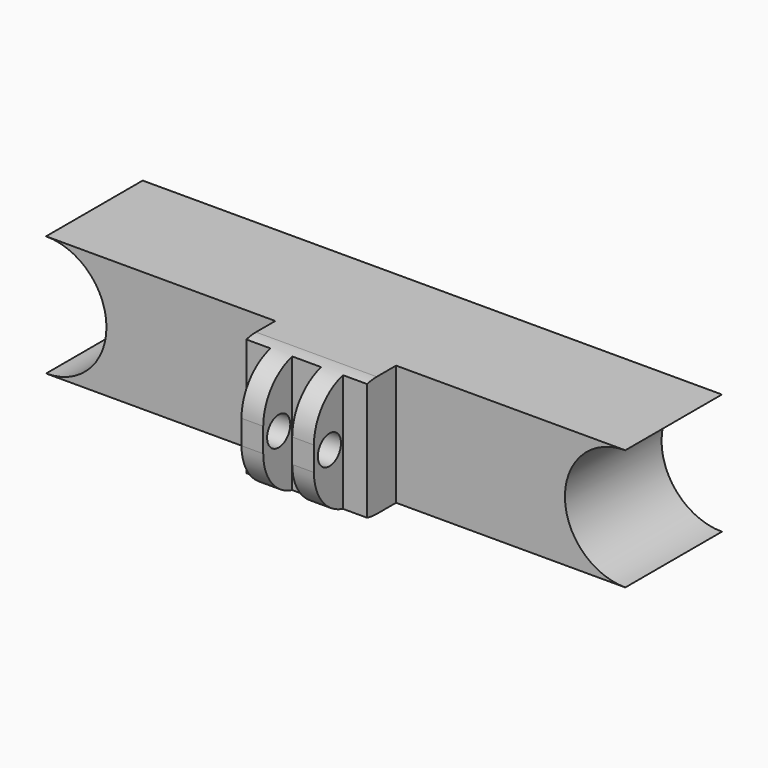
from build123d import *

# Parameters (mm, degrees)
F1_DEPTH  = 25
F2_W      = 50
F2_H      = 50
F3_DEPTH  = 30
F6_W      = 6
F6_H      = 15
F5_W      = 6
F5_H      = 15
F4_W      = 10
F4_H      = 15
F7_DEPTH  = 50.001
F8_F1_R   = 20
F8_F2_R   = 20
F9_R      = 6
F10_DEPTH = 134.901


with BuildPart() as f1:
    # F0 (on Front) → F1 (new body, symmetric)
    with BuildSketch(Plane.XZ):
        with BuildLine():
            Line((-119.9, -25), (119.9, -25))
            ThreePointArc((119.9, -25), (94.9, 0), (119.9, 25))
            Line((119.9, 25), (-119.9, 25))
            ThreePointArc((-119.9, 25), (-94.9, 0), (-119.9, -25))
        make_face()
    extrude(amount=F1_DEPTH, both=True)

    # F2 (on face) → F3 (join)
    with BuildSketch(Plane.XZ.offset(25)):
        Rectangle(F2_W, F2_H)
    extrude(amount=F3_DEPTH)

    # F6 (on face) + F5 (on face) + F4 (on face) → F7 (cut, through all)
    with BuildSketch(Plane(origin=(0, 0, -25), x_dir=(1, 0, 0), z_dir=(0, 0, -1))):
        with Locations((-3, 47.5)):
            Rectangle(F6_W, F6_H)
    with BuildSketch(Plane(origin=(0, 0, -25), x_dir=(1, 0, 0), z_dir=(0, 0, -1))):
        with Locations((3, 47.5)):
            Rectangle(F5_W, F5_H)
    with BuildSketch(Plane(origin=(0, 0, -25), x_dir=(1, 0, 0), z_dir=(0, 0, -1))):
        with Locations((20, 47.5)):
            Rectangle(F4_W, F4_H)
        with Locations((-20, 47.5)):
            Rectangle(F4_W, F4_H)
    extrude(amount=-F7_DEPTH, mode=Mode.SUBTRACT)

    # F8: fillet of radius 20 on 4 edges, made by hand

    # F8_f1
    f8_f1_edges = [f1.edges().sort_by_distance(p)[0] for p in [
        (10.5, -55, 25),
    ]]
    fillet(f8_f1_edges, radius=F8_F1_R)

    # F8_f2
    f8_f2_edges = [f1.edges().sort_by_distance(p)[0] for p in [
        (10.5, -55, -25),
    ]]
    fillet(f8_f2_edges, radius=F8_F2_R)

    # F9 (on face) → F10 (cut, through all)
    with BuildSketch(Plane.YZ.offset(15)):
        with Locations((-47, 0)):
            Circle(F9_R)
    extrude(amount=-F10_DEPTH, mode=Mode.SUBTRACT)


solid = f1.part
